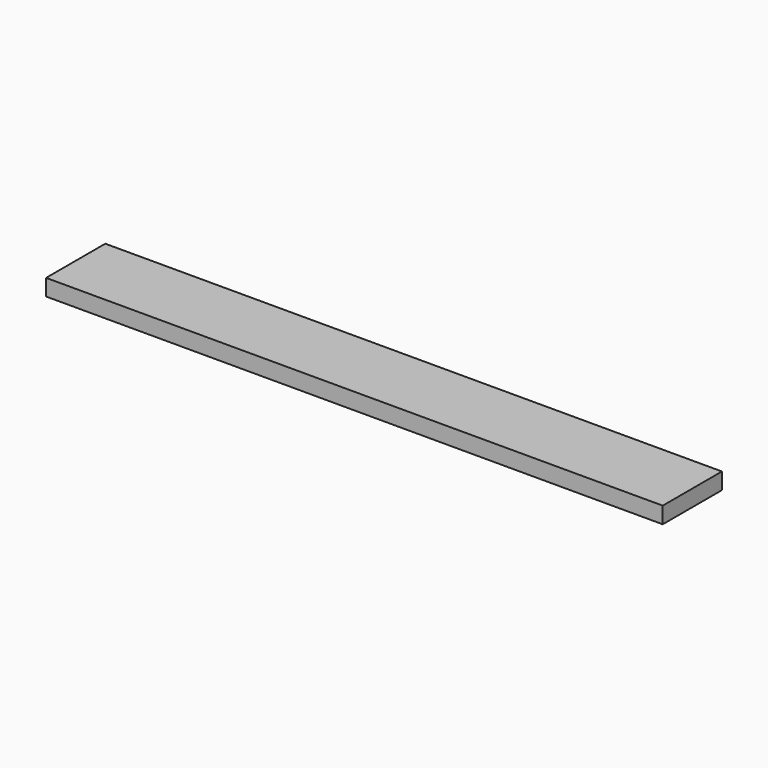
from build123d import *

# Parameters (mm, degrees)
F7_W     = 75
F7_H     = 9
F8_DEPTH = 2


# Not quite as in the source:
# - the program builds the solid bodies; features that only make, move or delete a surface that nothing else refers to are left out


with BuildPart() as f8:
    # F7 (on Top) → F8 (new body)
    with BuildSketch(Plane.XY):
        with Locations((0, 1.5)):
            Rectangle(F7_W, F7_H)
    extrude(amount=-F8_DEPTH)


solid = f8.part
